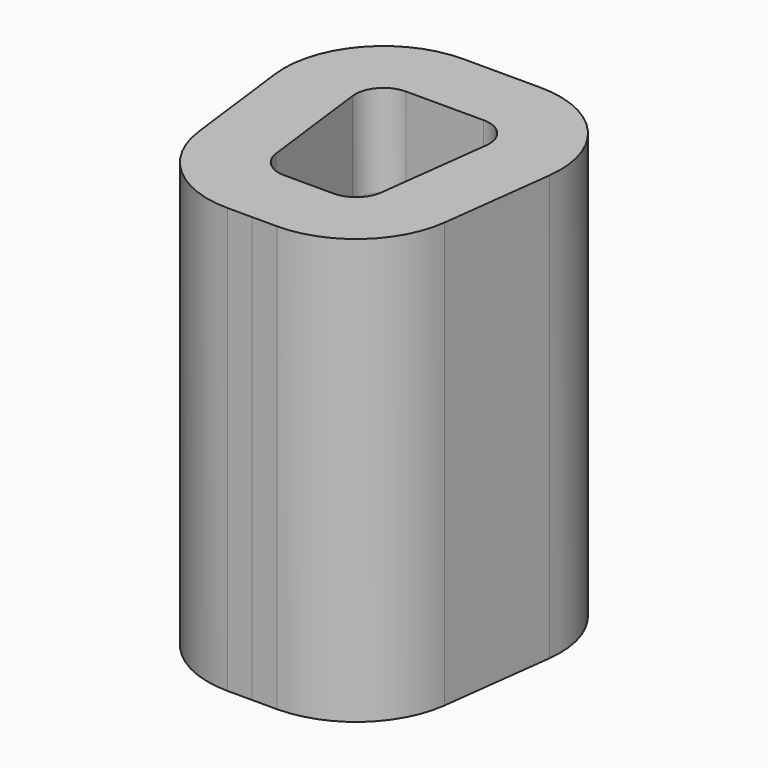
from build123d import *

# Parameters (mm, degrees)
F3_DEPTH = 30
F4_DEPTH = 8
F5_R     = 1.5


# Not quite as in the source:
# - ends of sketch curves that miss each other by under 0.0002 mm in the source are joined


with BuildPart() as f3:
    # F0 (on Top) → F3 (new body)
    with BuildSketch(Plane.XY):
        with BuildLine():
            Line((2.7344355629, 17), (0, 17))
            Line((0, 17), (-2.7344355629, 17))
            ThreePointArc((-2.7344355629, 17), (-7.9821831045, 14.6326182171), (-9.6803811114, 9.1317568064))
            Line((-9.6803811114, 9.1317568064), (-8.6803809552, 1.131756826))
            ThreePointArc((-8.6803809552, 1.131756826), (-6.3670534302, -3.2477471454), (-1.7344355629, -4.9999998862))
            Line((-1.7344355629, -4.9999998862), (0, -4.9999998882))
            Line((0, -4.9999998882), (1.7344355629, -5))
            ThreePointArc((1.7344355629, -5), (6.3670535056, -3.2477472307), (8.6803806999, 1.1317568579))
            Line((8.6803806999, 1.1317568579), (9.6803806999, 9.1317568579))
            ThreePointArc((9.6803806999, 9.1317568579), (7.9821826424, 14.6326178092), (2.7344355629, 17))
        make_face()
        with BuildLine():
            Line((1.7344355629, 0), (0, 0))
            Line((0, 0), (-1.7344355629, 0))
            ThreePointArc((-1.7344355629, 0), (-3.0580406894, 0.5006436484), (-3.7189913164, 1.7519305308))
            Line((-3.7189913164, 1.7519305308), (-4.7189913164, 9.7519305308))
            ThreePointArc((-4.7189913164, 9.7519305308), (-4.2337919146, 11.3236051265), (-2.7344355629, 12))
            Line((-2.7344355629, 12), (0, 12))
            Line((0, 12), (2.7344355629, 12))
            ThreePointArc((2.7344355629, 12), (4.2337919146, 11.3236051265), (4.7189913164, 9.7519305308))
            Line((4.7189913164, 9.7519305308), (3.7189913164, 1.7519305308))
            ThreePointArc((3.7189913164, 1.7519305308), (3.0580406894, 0.5006436484), (1.7344355629, 0))
        make_face(mode=Mode.SUBTRACT)
        with BuildLine():
            Line((-1.7344355629, 0), (0, 0))
            Line((0, 0), (0, 3))
            ThreePointArc((0, 3), (-3, 6), (0, 9))
            Line((0, 9), (0, 12))
            Line((0, 12), (-2.7344355629, 12))
            ThreePointArc((-2.7344355629, 12), (-4.2337919146, 11.3236051265), (-4.7189913164, 9.7519305308))
            Line((-4.7189913164, 9.7519305308), (-3.7189913164, 1.7519305308))
            ThreePointArc((-3.7189913164, 1.7519305308), (-3.0580406894, 0.5006436484), (-1.7344355629, 0))
        make_face()
        with BuildLine():
            Line((0, 3), (0, 0))
            Line((0, 0), (1.7344355629, 0))
            ThreePointArc((1.7344355629, 0), (3.0580406894, 0.5006436484), (3.7189913164, 1.7519305308))
            Line((3.7189913164, 1.7519305308), (4.7189913164, 9.7519305308))
            ThreePointArc((4.7189913164, 9.7519305308), (4.2337919146, 11.3236051265), (2.7344355629, 12))
            Line((2.7344355629, 12), (0, 12))
            Line((0, 12), (0, 9))
            ThreePointArc((0, 9), (2.1213203436, 8.1213203436), (3, 6))
            ThreePointArc((3, 6), (2.1213203436, 3.8786796564), (0, 3))
        make_face()
    extrude(amount=F3_DEPTH)

    # F2 (on offset) → F4 (cut)
    with BuildSketch(Plane.XY.offset(30)):
        with BuildLine():
            ThreePointArc((-3.7189913164, 1.7519305308), (-3.0580406894, 0.5006436484), (-1.7344355629, 0))
            Line((-1.7344355629, 0), (0, 0))
            Line((0, 0), (0, 3))
            ThreePointArc((0, 3), (-3, 6), (0, 9))
            Line((0, 9), (0, 12))
            Line((0, 12), (-2.7344355629, 12))
            ThreePointArc((-2.7344355629, 12), (-4.2337919146, 11.3236051265), (-4.7189913164, 9.7519305308))
            Line((-4.7189913164, 9.7519305308), (-3.7189913164, 1.7519305308))
        make_face()
        with BuildLine():
            Line((0, 3), (0, 0))
            Line((0, 0), (1.7344355629, 0))
            ThreePointArc((1.7344355629, 0), (3.0580406894, 0.5006436484), (3.7189913164, 1.7519305308))
            Line((3.7189913164, 1.7519305308), (4.7189913164, 9.7519305308))
            ThreePointArc((4.7189913164, 9.7519305308), (4.2337919146, 11.3236051265), (2.7344355629, 12))
            Line((2.7344355629, 12), (0, 12))
            Line((0, 12), (0, 9))
            ThreePointArc((0, 9), (3, 6), (0, 3))
        make_face()
    extrude(amount=-F4_DEPTH, mode=Mode.SUBTRACT)

    # F5
    f5_edges = [f3.edges().sort_by_distance(p)[0] for p in [
        (-4.233792, 11.323605, 22),
        (-4.218991, 5.751931, 22),
    ]]
    fillet(f5_edges, radius=F5_R)


solid = f3.part
